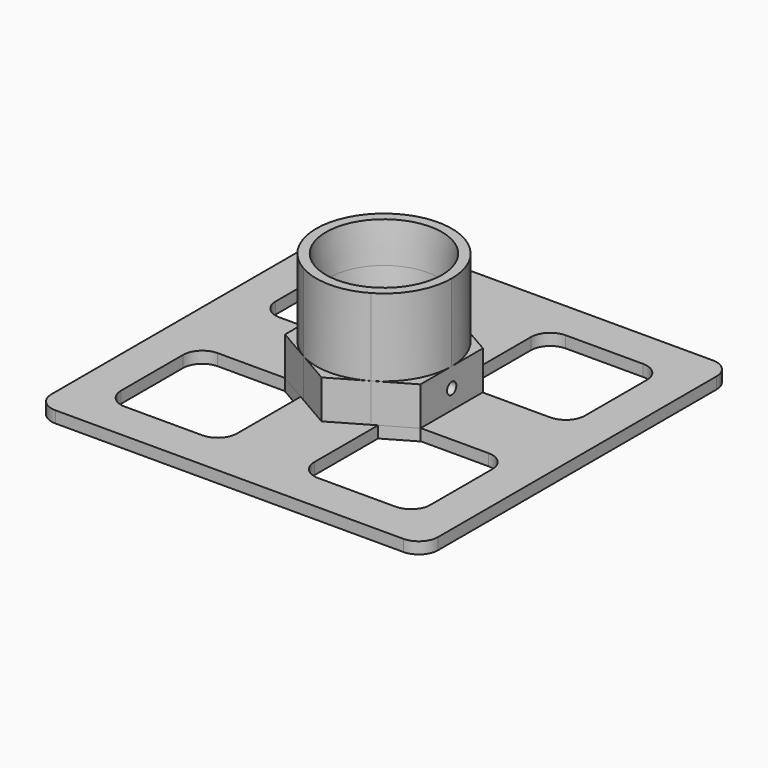
from build123d import *

# Parameters (mm, degrees)
F0_R      = 2.6
F1_DEPTH  = 10
F2_R      = 14
F3_DEPTH  = 20
F4_R      = 1.5
F5_DEPTH  = 35.001
F6_SIZE2  = 0.99999
F6_SIZE   = 9.99999
F7_W      = 100
F7_H      = 100
F8_DEPTH  = 3
F10_DEPTH = 25
F11_R     = 5


# Not quite as in the source:
# - a fillet or chamfer is up to 0.001 mm smaller than in the source, because OpenCascade refuses the exact size


with BuildPart() as f1:
    # F0 (on Top) → F1 (new body)
    with BuildSketch(Plane.XY):
        with BuildLine():
            ThreePointArc((8.7499999554, -15.155444592), (15.1554445533, -8.7500000223), (17.5, 0))
            ThreePointArc((17.5, 0), (15.15544445, 8.7500002013), (8.7499995974, 15.1554447987))
            ThreePointArc((8.7499995974, 15.1554447987), (-2.067e-07, 17.5), (-8.7499999554, 15.155444592))
            ThreePointArc((-8.7499999554, 15.155444592), (-15.155444558, 8.7500000142), (-17.5, -1.86e-08))
            ThreePointArc((-17.5, -1.86e-08), (-15.1554444739, -8.7500001599), (-8.7499996963, -15.1554447416))
            ThreePointArc((-8.7499996963, -15.1554447416), (1.496e-07, -17.5), (8.7499999554, -15.155444592))
        make_face()
        Circle(F0_R, mode=Mode.SUBTRACT)
        with BuildLine():
            Line((-17.5, -10.1036297108), (-8.7499996963, -15.1554447416))
            ThreePointArc((-8.7499996963, -15.1554447416), (-15.1554444739, -8.7500001599), (-17.5, -1.86e-08))
            Line((-17.5, -1.86e-08), (-17.5, -10.1036297108))
        make_face()
        with BuildLine():
            Line((0, -20.2072594216), (8.7499999554, -15.155444592))
            ThreePointArc((8.7499999554, -15.155444592), (1.496e-07, -17.5), (-8.7499996963, -15.1554447416))
            Line((-8.7499996963, -15.1554447416), (0, -20.2072594216))
        make_face()
        with BuildLine():
            Line((17.5, -10.1036297108), (17.5, 0))
            ThreePointArc((17.5, 0), (15.1554445533, -8.7500000223), (8.7499999554, -15.155444592))
            Line((8.7499999554, -15.155444592), (17.5, -10.1036297108))
        make_face()
        with BuildLine():
            ThreePointArc((8.7499995974, 15.1554447987), (15.15544445, 8.7500002013), (17.5, 0))
            Line((17.5, 0), (17.5, 10.1036297108))
            Line((17.5, 10.1036297108), (8.7499995974, 15.1554447987))
        make_face()
        with BuildLine():
            ThreePointArc((-8.7499999554, 15.155444592), (-2.067e-07, 17.5), (8.7499995974, 15.1554447987))
            Line((8.7499995974, 15.1554447987), (0, 20.2072594216))
            Line((0, 20.2072594216), (-8.7499999554, 15.155444592))
        make_face()
        with BuildLine():
            ThreePointArc((-17.5, -1.86e-08), (-15.155444558, 8.7500000142), (-8.7499999554, 15.155444592))
            Line((-8.7499999554, 15.155444592), (-17.5, 10.1036297108))
            Line((-17.5, 10.1036297108), (-17.5, -1.86e-08))
        make_face()
    extrude(amount=F1_DEPTH)

    # F2 (on face) → F3 (join)
    with BuildSketch(Plane.XY.offset(10)):
        with BuildLine():
            ThreePointArc((8.7500002145, -15.1554444424), (15.1554446281, -8.7499998928), (17.5, 0))
            ThreePointArc((17.5, 0), (15.1554446281, 8.7499998928), (8.7500002145, 15.1554444424))
            ThreePointArc((8.7500002145, 15.1554444424), (1.496e-07, 17.5), (-8.7499999554, 15.155444592))
            ThreePointArc((-8.7499999554, 15.155444592), (-15.155444558, 8.7500000142), (-17.5, -1.86e-08))
            ThreePointArc((-17.5, -1.86e-08), (-15.1554446126, -8.7499999197), (-8.7500001767, -15.1554444642))
            ThreePointArc((-8.7500001767, -15.1554444642), (2.18e-08, -17.5), (8.7500002145, -15.1554444424))
        make_face()
        Circle(F2_R, mode=Mode.SUBTRACT)
    extrude(amount=F3_DEPTH)

    # F4 (on face) → F5 (cut, through all)
    with BuildSketch(Plane(origin=(-17.5, 0, 0), x_dir=(0, -1, 0), z_dir=(-1, 0, 0))):
        with Locations((0, 5)):
            Circle(F4_R)
    extrude(amount=-F5_DEPTH, mode=Mode.SUBTRACT)

    # F6 (size 10 and 1 in the source; OpenCascade refuses exactly that, so slightly less here)
    f6_edges = [f1.edges().sort_by_distance(p)[0] for p in [
        (14, 0, 20),
        (-14, 0, 10),
        (-14, 0, 30),
    ]]
    f6_side = f1.faces().sort_by_distance((-14, 0, 20))[0]
    chamfer(f6_edges, length=F6_SIZE, length2=F6_SIZE2, reference=f6_side)

    # F7 (on Top) → F8 (join)
    with BuildSketch(Plane.XY):
        Rectangle(F7_W, F7_H)
    extrude(amount=-F8_DEPTH)

    # F9 (on face) → F10 (cut)
    with BuildSketch(Plane.XY):
        Polygon((-40, 40), (-40, 10), (-17.5, 10), (-17.5, 10.1036297108), (-10, 14.4337567297), (-10, 40), align=None)
        Polygon((17.5, 10), (40, 10), (40, 40), (10, 40), (10, 14.4337567297), (17.5, 10.1036297108), align=None)
        Polygon((10, -14.4337567297), (10, -40), (40, -40), (40, -10), (17.5, -10), (17.5, -10.1036297108), align=None)
        Polygon((-40, -10), (-40, -40), (-10, -40), (-10, -14.4337567297), (-17.5, -10.1036297108), (-17.5, -10), align=None)
    extrude(amount=-F10_DEPTH, mode=Mode.SUBTRACT)

    # F11
    f11_edges = [f1.edges().sort_by_distance(p)[0] for p in [
        (-40, 40, -1.5),
        (-10, 40, -1.5),
        (-40, 10, -1.5),
        (10, 40, -1.5),
        (40, 40, -1.5),
        (40, 10, -1.5),
        (40, -10, -1.5),
        (10, -40, -1.5),
        (40, -40, -1.5),
        (-10, -40, -1.5),
        (-40, -40, -1.5),
        (-40, -10, -1.5),
        (50, -50, -1.5),
        (-50, -50, -1.5),
        (-50, 50, -1.5),
        (50, 50, -1.5),
    ]]
    fillet(f11_edges, radius=F11_R)


solid = f1.part
